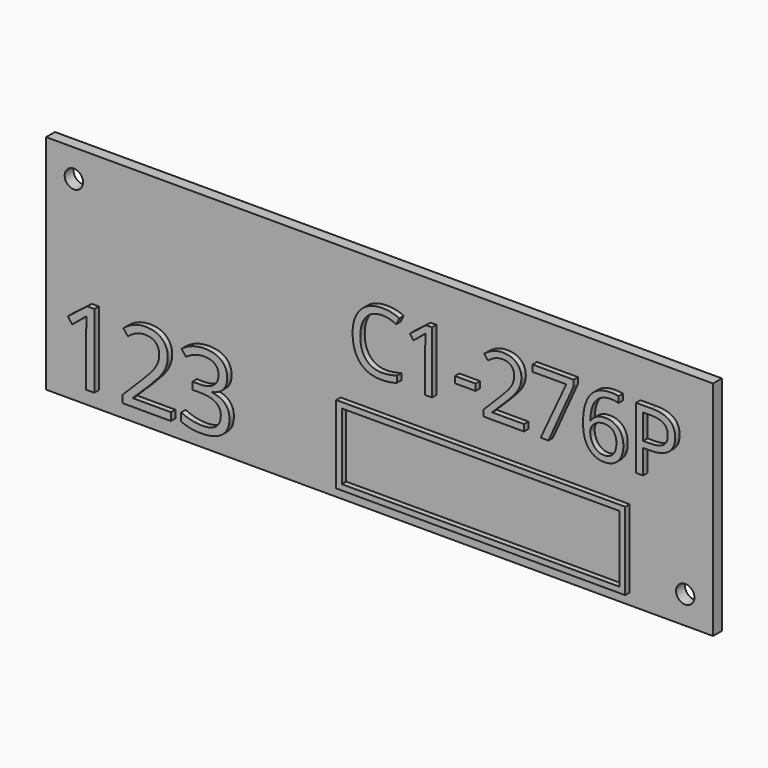
from build123d import *

# Parameters (mm, degrees)
F0_W         = 120
F0_H         = 40
F1_DEPTH     = 2
F3_D         = 3.3
F4_TEXT_SIZE = 15.5635715154
F5_DEPTH     = 1
F6_TEXT_SIZE = 18.5894526641
F7_DEPTH     = 1
F8_W         = 52
F8_H         = 14
F8_W_2       = 49.99999962
F8_H_2       = 11.99999962
F9_DEPTH     = 1


# Not quite as in the source:
# - Text() gives the source's letters only with a copy of the font that has no kerning and outlines rounded to 1/6400 em; it was checked with that copy


with BuildPart() as f1:
    # F0 (on Front) → F1 (new body)
    with BuildSketch(Plane.XZ):
        Rectangle(F0_W, F0_H)
    extrude(amount=F1_DEPTH)

    # F3 (through all)
    with Locations(Plane.XZ.offset(2)):
        with Locations((-55, 15), (55, -15)):
            Hole(F3_D / 2)

    # F4 (on face) → F5 (join)
    with BuildSketch(Plane.XZ.offset(2)):
        with Locations((-5, 2)):
            Text('C1-276P', F4_TEXT_SIZE, font='Open Sans', text_align=(TextAlign.LEFT, TextAlign.BOTTOM))
    extrude(amount=F5_DEPTH)

    # F6 (on face) → F7 (join)
    with BuildSketch(Plane.XZ.offset(2)):
        with Locations((-57, -17)):
            Text('123', F6_TEXT_SIZE, font='Open Sans', text_align=(TextAlign.LEFT, TextAlign.BOTTOM))
    extrude(amount=F7_DEPTH)

    # F8 (on face) → F9 (join)
    with BuildSketch(Plane.XZ.offset(2)):
        with Locations((19, -11)):
            Rectangle(F8_W, F8_H)
        with Locations((19, -11)):
            Rectangle(F8_W_2, F8_H_2, mode=Mode.SUBTRACT)
    extrude(amount=F9_DEPTH)


solid = f1.part
